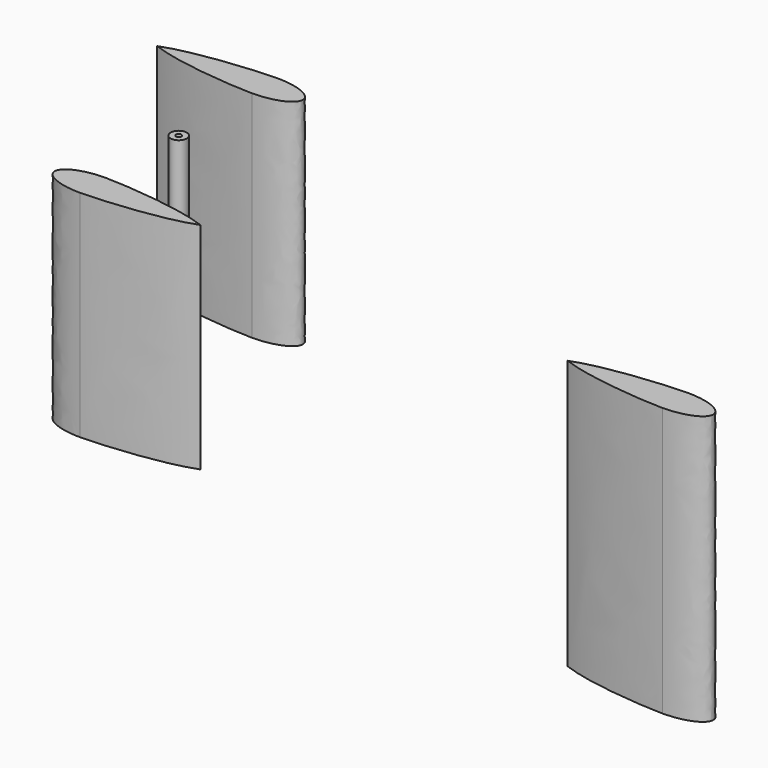
from build123d import *

# Parameters (mm, degrees)
F1_DEPTH = 250
F2_DEPTH = 200
F0_R     = 7.5
F0_R_2   = 2.5


# Not quite as in the source:
# - ends of sketch curves that miss each other by under 0.0002 mm in the source are joined
# - the program builds the solid bodies; features that only make, move or delete a surface that nothing else refers to are left out


with BuildPart() as f1:
    # F0 (on Top) → F1 (new body)
    with BuildSketch(Plane.XY):
        with BuildLine():
            add(Edge.make_bspline(
                [(0, -15), (35.3319384158, -15), (35.3319384158, 0), (35.3319384158, 15), (0, 15)],
                knots=[1.5707963268, 1.5707963268, 1.5707963268, 3.1415926536, 3.1415926536, 4.7123889804, 4.7123889804, 4.7123889804], degree=2, weights=[1, 0.7071067812, 1, 0.7071067812, 1]))
            add(Edge.make_bspline(
                [(0, 15), (-16.2319140521, 15.0000000963), (-71.5773864947, 10.9885398261), (-100.0000014291, -1.909e-07)],
                knots=[0, 0, 0, 0, 101.1187435224, 101.1187435224, 101.1187435224, 101.1187435224], degree=3))
            add(Edge.make_bspline(
                [(0, -15), (-16.2319140521, -15.0000000963), (-71.5773864947, -10.9885398261), (-100.0000014291, -1.909e-07)],
                knots=[0, 0, 0, 0, 101.1187435224, 101.1187435224, 101.1187435224, 101.1187435224], degree=3))
        make_face()
    extrude(amount=-F1_DEPTH)


with BuildPart() as f2:
    # F0 (on Top) → F2 (new body)
    with BuildSketch(Plane.XY):
        with BuildLine():
            add(Edge.make_bspline(
                [(-301.4754507362, -114.9492457264), (-266.1435123205, -114.9492457264), (-266.1435123205, -99.9492457264), (-266.1435123205, -84.9492457264), (-301.4754507362, -84.9492457264)],
                knots=[1.5707963268, 1.5707963268, 1.5707963268, 3.1415926536, 3.1415926536, 4.7123889804, 4.7123889804, 4.7123889804], degree=2, weights=[1, 0.7071067812, 1, 0.7071067812, 1]))
            add(Edge.make_bspline(
                [(-301.4754507362, -84.9492457264), (-317.7073647883, -84.9492456301), (-373.0528372309, -88.9607059003), (-401.4754521653, -99.9492459173)],
                knots=[0, 0, 0, 0, 101.1187435224, 101.1187435224, 101.1187435224, 101.1187435224], degree=3))
            add(Edge.make_bspline(
                [(-301.4754507362, -114.9492457264), (-317.7073647883, -114.9492458228), (-373.0528372309, -110.9377855526), (-401.4754521653, -99.9492459173)],
                knots=[0, 0, 0, 0, 101.1187435224, 101.1187435224, 101.1187435224, 101.1187435224], degree=3))
        make_face()
    extrude(amount=F2_DEPTH)


with BuildPart() as f2b:
    # F0 (on Top) → F2, piece 2 (new body)
    with BuildSketch(Plane.XY):
        with BuildLine():
            add(Edge.make_bspline(
                [(-301.3535811887, -284.9492457264), (-285.1216671366, -284.9492456301), (-229.776194694, -288.9607059003), (-201.3535797596, -299.9492459173)],
                knots=[0, 0, 0, 0, 101.1187435224, 101.1187435224, 101.1187435224, 101.1187435224], degree=3))
            add(Edge.make_bspline(
                [(-301.3535811887, -284.9492457264), (-336.6855196045, -284.9492457264), (-336.6855196045, -299.9492457264), (-336.6855196045, -314.9492457264), (-301.3535811887, -314.9492457264)],
                knots=[4.7123889804, 4.7123889804, 4.7123889804, 6.2831853072, 6.2831853072, 7.853981634, 7.853981634, 7.853981634], degree=2, weights=[1, 0.7071067812, 1, 0.7071067812, 1]))
            add(Edge.make_bspline(
                [(-301.3535811887, -314.9492457264), (-285.1216671366, -314.9492458228), (-229.776194694, -310.9377855526), (-201.3535797596, -299.9492459173)],
                knots=[0, 0, 0, 0, 101.1187435224, 101.1187435224, 101.1187435224, 101.1187435224], degree=3))
        make_face()
    extrude(amount=F2_DEPTH)


with BuildPart() as f2c:
    # F0 (on Top) → F2, piece 3 (new body)
    with BuildSketch(Plane.XY):
        with Locations((-301.4754507362, -199.9492457264)):
            Circle(F0_R)
        with Locations((-301.4754507362, -199.9492457264)):
            Circle(F0_R_2, mode=Mode.SUBTRACT)
    extrude(amount=F2_DEPTH)


solid = Compound([f1.part, f2.part, f2b.part, f2c.part])
